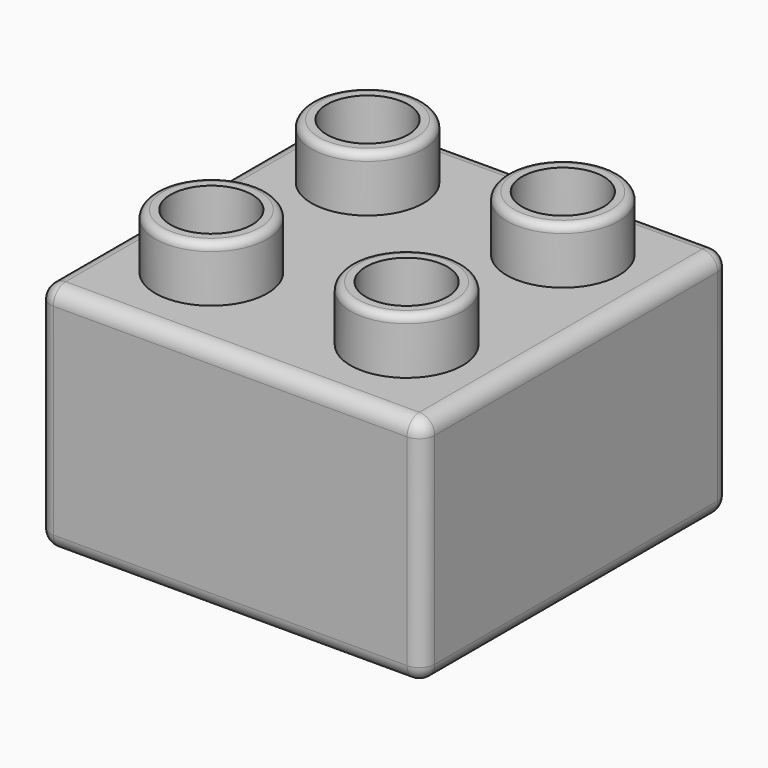
from build123d import *

# Parameters (mm, degrees)
F0_W          = 31.75
F0_H          = 31.75
F5_DEPTH      = 19.177
F1_W          = 28.575
F1_H          = 28.575
F6_DEPTH      = 18.161
F6_DEPTH_BACK = 0.381
F2_R          = 6.5405
F7_DEPTH      = 15.875
F3_R          = 5.461
F8_DEPTH      = 15.875
F8_DEPTH_BACK = 0.635
F4_W          = 1.016
F4_H          = 2.286
F10_DEPTH     = 17.526
F15_ANGLE     = 90
F16_R         = 4.6355
F18_DEPTH     = 4.699
F17_R         = 3.3655
F19_DEPTH     = 4.699
F23_R         = 1.26999
F24_R         = 0.635
F24_2_R       = 0.635
F24_3_R       = 0.635
F24_4_R       = 0.635


# Not quite as in the source:
# - a fillet or chamfer is up to 0.001 mm smaller than in the source, because OpenCascade refuses the exact size


with BuildPart() as f5:
    # F0 (on Top) → F5 (new body)
    with BuildSketch(Plane.XY):
        with Locations((0, -0.3175)):
            Rectangle(F0_W, F0_H)
    extrude(amount=F5_DEPTH)

    # F1 (on face) → F6 (cut, two sides)
    with BuildSketch(Plane.XY) as f6_sk:
        Rectangle(F1_W, F1_H)
    extrude(amount=F6_DEPTH, mode=Mode.SUBTRACT)
    extrude(f6_sk.sketch, amount=-F6_DEPTH_BACK, mode=Mode.SUBTRACT)

    # F23 (radius 1.27 in the source; OpenCascade refuses exactly that, so slightly less here)
    f23_edges = [f5.edges().sort_by_distance(p)[0] for p in [
        (0, -16.1925, 19.177),
        (-15.875, -0.3175, 19.177),
        (0, 15.5575, 19.177),
        (15.875, -0.3175, 19.177),
        (-15.875, -16.1925, 9.5885),
        (15.875, -16.1925, 9.5885),
        (-15.875, 15.5575, 9.5885),
        (15.875, 15.5575, 9.5885),
        (15.875, -0.3175, 0),
        (0, -16.1925, 0),
        (-15.875, -0.3175, 0),
        (0, 15.5575, 0),
    ]]
    fillet(f23_edges, radius=F23_R)


with BuildPart() as f7:
    # F2 (on face) → F7 (new body)
    with BuildSketch(Plane.XY):
        Circle(F2_R)
    extrude(amount=F7_DEPTH)

    # F3 (on face) → F8 (cut, two sides)
    with BuildSketch(Plane.XY) as f8_sk:
        Circle(F3_R)
    extrude(amount=F8_DEPTH, mode=Mode.SUBTRACT)
    extrude(f8_sk.sketch, amount=-F8_DEPTH_BACK, mode=Mode.SUBTRACT)


with BuildPart() as f7_1:
    # F9: moved
    add(f7.part.moved(Location((0, 0, 2.286))))


with BuildPart() as f10:
    # F4 (on face) → F10 (new body)
    with BuildSketch(Plane.XY):
        with Locations((0, -0.357)):
            Rectangle(F4_W, F4_H)
    extrude(amount=F10_DEPTH)


with BuildPart() as f10_1:
    # F11: moved
    add(f10.part.moved(Location((8.0645, 13.8557, 0.635))))


with BuildPart() as f12_1:
    # F12: instance of F10
    add(f10_1.part.mirror(Plane.XZ))


with BuildPart() as f13_1:
    # F13: instance of F12_1
    add(f12_1.part.mirror(Plane.YZ))


with BuildPart() as f13_2:
    # F13: instance of F10
    add(f10_1.part.mirror(Plane.YZ))


with BuildPart() as f15_1:
    # F15: copy of F12_1
    add(f12_1.part.rotate(Axis((0, 0, 4.273429513), (0, 0, -1)), F15_ANGLE))


with BuildPart() as f15_2:
    # F15: copy of F13_1
    add(f13_1.part.rotate(Axis((0, 0, 4.273429513), (0, 0, -1)), F15_ANGLE))


with BuildPart() as f15_3:
    # F15: copy of F10
    add(f10_1.part.rotate(Axis((0, 0, 4.273429513), (0, 0, -1)), F15_ANGLE))


with BuildPart() as f15_4:
    # F15: copy of F13_2
    add(f13_2.part.rotate(Axis((0, 0, 4.273429513), (0, 0, -1)), F15_ANGLE))


with BuildPart() as f18:
    # F16 (on Top) → F18 (new body)
    with BuildSketch(Plane.XY):
        Circle(F16_R)
    extrude(amount=F18_DEPTH)

    # F17 (on Top) → F19 (cut)
    with BuildSketch(Plane.XY):
        Circle(F17_R)
    extrude(amount=F19_DEPTH, mode=Mode.SUBTRACT)


with BuildPart() as f18_1:
    # F20: moved
    add(f18.part.moved(Location((8.0645, 8.0645, 19.05))))


with BuildPart() as f21_1:
    # F21: instance of F18
    add(f18_1.part.mirror(Plane.XZ))


with BuildPart() as f22_1:
    # F22: instance of F18
    add(f18_1.part.mirror(Plane.YZ))

    # F24
    f24_edges = [f22_1.edges().sort_by_distance(p)[0] for p in [
        (-3.429, 8.0645, 23.749),
    ]]
    fillet(f24_edges, radius=F24_R)


with BuildPart() as f22_2:
    # F22: instance of F21_1
    add(f21_1.part.mirror(Plane.YZ))

    # F24#4
    f24_4_edges = [f22_2.edges().sort_by_distance(p)[0] for p in [
        (-3.429, -8.0645, 23.749),
    ]]
    fillet(f24_4_edges, radius=F24_4_R)


with BuildPart() as f18_2:
    add(f18_1.part)

    # F24#2
    f24_2_edges = [f18_2.edges().sort_by_distance(p)[0] for p in [
        (3.429, 8.0645, 23.749),
    ]]
    fillet(f24_2_edges, radius=F24_2_R)


with BuildPart() as f21_1_1:
    add(f21_1.part)

    # F24#3
    f24_3_edges = [f21_1_1.edges().sort_by_distance(p)[0] for p in [
        (3.429, -8.0645, 23.749),
    ]]
    fillet(f24_3_edges, radius=F24_3_R)


solid = Compound([f5.part, f7_1.part, f10_1.part, f12_1.part, f13_1.part, f13_2.part, f15_1.part, f15_2.part, f15_3.part, f15_4.part, f22_1.part, f22_2.part, f18_2.part, f21_1_1.part])
